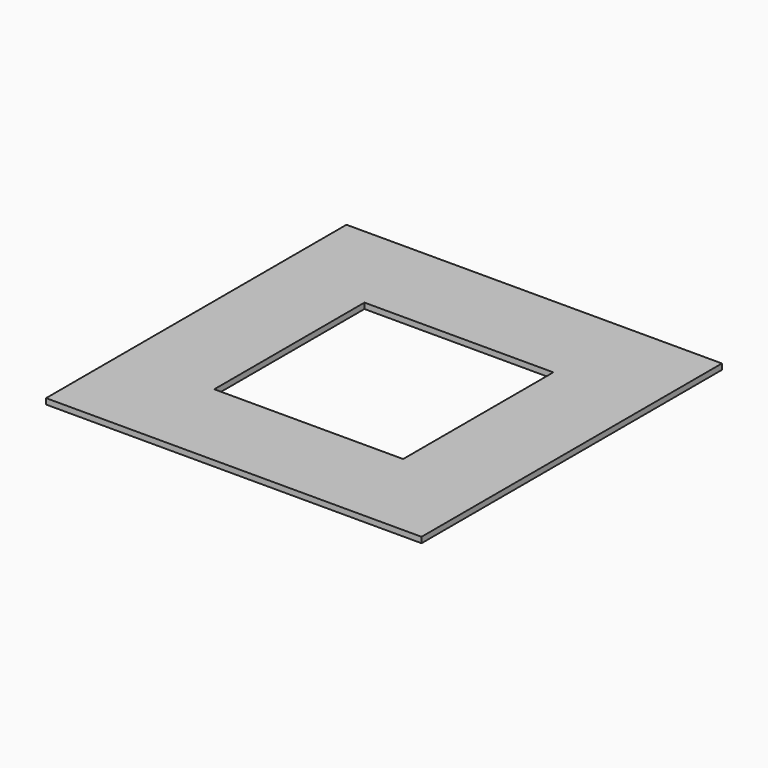
from build123d import *

# Parameters (mm, degrees)
F0_W     = 838.2
F0_H     = 838.2
F1_DEPTH = 12.7
F2_W     = 421.64
F2_H     = 419.1
F3_DEPTH = 25.4


# Not quite as in the source:
# - a length typed as a fraction of an inch, garbled in the dataset ("3 / 203.2 mm" for 3/8 in), is restored


with BuildPart() as f1:
    # F0 (on Top) → F1 (new body)
    with BuildSketch(Plane.XY):
        with Locations((-8.0585610121, 9.1306694565)):
            Rectangle(F0_W, F0_H)
    extrude(amount=F1_DEPTH)

    # F2 (on face) → F3 (cut)
    with BuildSketch(Plane.XY.offset(12.7)):
        with Locations((-8.2721859217, 8.8253611648)):
            Rectangle(F2_W, F2_H)
    extrude(amount=-F3_DEPTH, mode=Mode.SUBTRACT)


solid = f1.part
